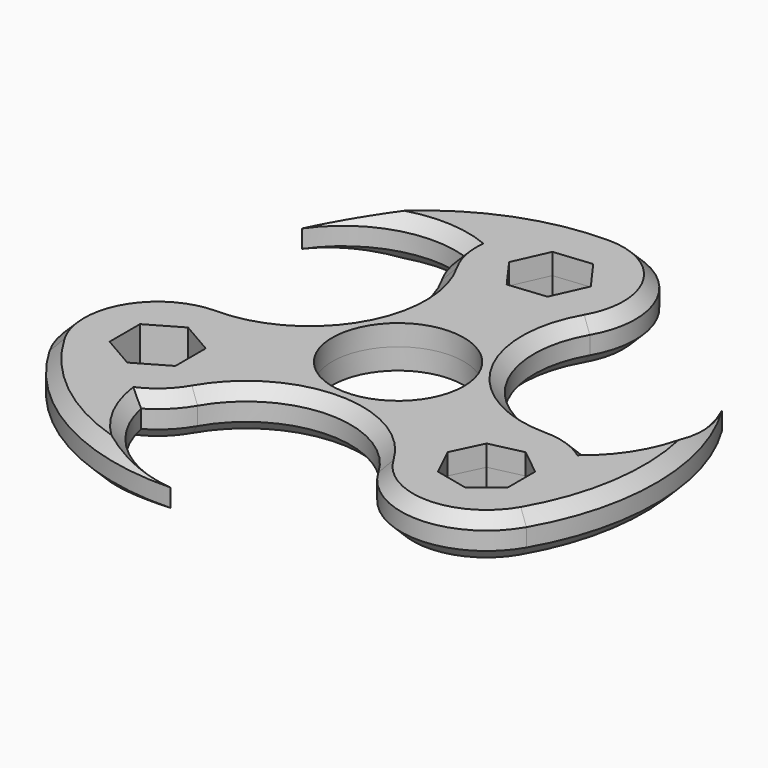
from build123d import *

# Parameters (mm, degrees)
F0_R          = 11
F1_DEPTH      = 3.5
F1_DEPTH_BACK = 3.5
F2_SIZE       = 2


# Not quite as in the source:
# - a feature names something its author has since deleted; it is built from what else it names


with BuildPart() as f1:
    # F0 (on Top) → F1 (new body, two sides)
    with BuildSketch(Plane.XY) as f1_sk:
        with BuildLine():
            ThreePointArc((-36.7798490863, 25.1142671396), (-27.219118588, 32.264950132), (-15.2801158302, 32.2580171396))
            ThreePointArc((-15.2801158302, 32.2580171396), (-14.7932810733, 28.5601400327), (-13.3659537868, 25.1142671396))
            ThreePointArc((-13.3659537868, 25.1142671396), (-13.3659537868, 7.6517671396), (-28.4889224003, -1.0794828604))
            ThreePointArc((-28.4889224003, -1.0794828604), (-40.8622603569, -8.2232328604), (-40.8622603569, -22.5107328604))
            ThreePointArc((-40.8622603569, -22.5107328604), (-25.4390445698, -37.6894940637), (-4.408636794, -42.7877609913))
            ThreePointArc((-4.408636794, -42.7877609913), (-15.3816751689, -38.0832669973), (-21.3451724003, -27.740320817))
            ThreePointArc((-21.3451724003, -27.740320817), (-18.3861342641, -25.4697709966), (-16.1155844438, -22.5107328604))
            ThreePointArc((-16.1155844438, -22.5107328604), (-0.9926158302, -13.7794828604), (14.1303527834, -22.5107328604))
            ThreePointArc((14.1303527834, -22.5107328604), (26.50369074, -29.6544828604), (38.8770286965, -22.5107328604))
            ThreePointArc((38.8770286965, -22.5107328604), (44.310613603, -1.5644555791), (38.2106383897, 19.1975452705))
            ThreePointArc((38.2106383897, 19.1975452705), (39.6229462664, 7.3423682841), (33.64744074, -2.9936449038))
            ThreePointArc((33.64744074, -2.9936449038), (30.2015678469, -1.5663176173), (26.50369074, -1.0794828604))
            ThreePointArc((26.50369074, -1.0794828604), (11.3807221264, 7.6517671396), (11.3807221264, 25.1142671396))
            ThreePointArc((11.3807221264, 25.1142671396), (11.3807221264, 39.4017671396), (-0.9926158302, 46.5455171396))
            ThreePointArc((-0.9926158302, 46.5455171396), (-21.8494165238, 40.7780010616), (-36.7798490863, 25.1142671396))
        make_face()
        Polygon((-28.4889224003, -21.7169828604), (-33.9881837144, -18.5419828604), (-33.9881837144, -12.1919828604), (-28.4889224003, -9.0169828604), (-22.9896610863, -12.1919828604), (-22.9896610863, -18.5419828604), align=None, mode=Mode.SUBTRACT)
        with Locations((-0.9926158302, 0.5080171396)):
            Circle(F0_R, mode=Mode.SUBTRACT)
        Polygon((27.9530368024, -9.0169828604), (32.3719731429, -12.5409669992), (32.3719731429, -18.1929987216), (27.9530368024, -21.7169828604), (22.4427133156, -20.4592874828), (19.9903886582, -15.3669828604), (22.4427133156, -10.274678238), align=None, mode=Mode.SUBTRACT)
        Polygon((5.3248489637, 32.8999973403), (2.7220877293, 27.1079222409), (-3.5953770646, 26.4659420402), (-5.1476309604, 28.6179993288), (-7.3100806241, 31.6160369389), (-4.7073193896, 37.4081120383), (1.6101454042, 38.050092239), align=None, mode=Mode.SUBTRACT)
    extrude(amount=F1_DEPTH)
    extrude(f1_sk.sketch, amount=-F1_DEPTH_BACK)

    # F2
    f2_edges = [f1.edges().sort_by_distance(p)[0] for p in [
        (-25.439045, -37.689494, 3.5),
        (-25.439045, -37.689494, -3.5),
        (-21.849417, 40.778001, -3.5),
        (-21.849417, 40.778001, 3.5),
        (26.503691, -29.654483, -3.5),
        (26.503691, -29.654483, 3.5),
        (-27.219119, 32.26495, 3.5),
        (39.622946, 7.342368, -3.5),
        (39.622946, 7.342368, 3.5),
        (-27.219119, 32.26495, -3.5),
        (-15.381675, -38.083267, -3.5),
        (-15.381675, -38.083267, 3.5),
    ]]
    chamfer(f2_edges, length=F2_SIZE)


solid = f1.part
